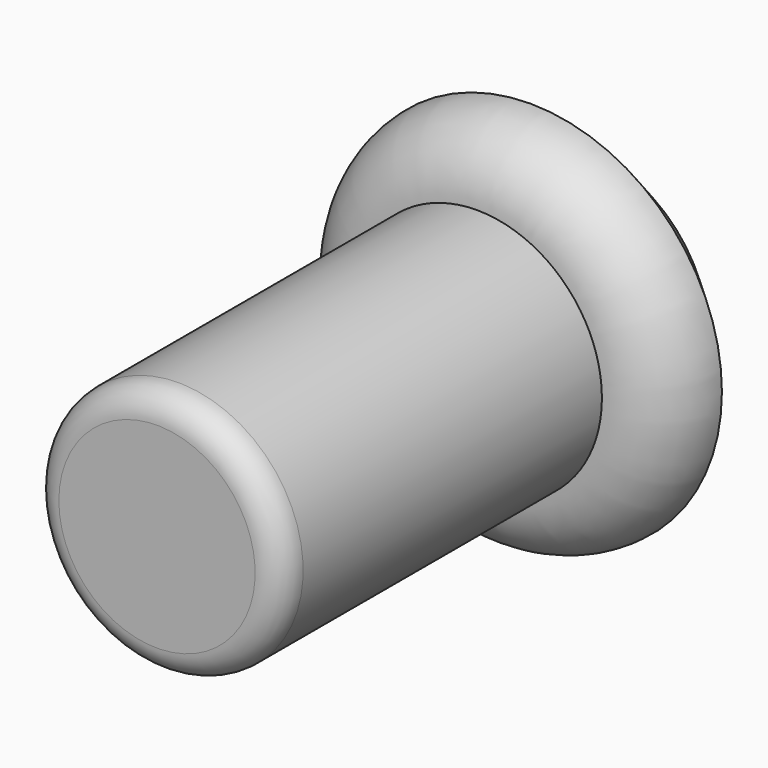
from build123d import *

# Parameters (mm, degrees)
F1_R     = 36.4721508719
F2_DEPTH = 25.399999693
F3_SIZE  = 12.7
F4_R     = 12.69999
F5_R     = 23.7721508719
F6_DEPTH = 101.6
F7_R     = 5.08


# Not quite as in the source:
# - a fillet or chamfer is up to 0.001 mm smaller than in the source, because OpenCascade refuses the exact size


with BuildPart() as f2:
    # F1 (on face) → F2 (new body)
    with BuildSketch(Plane.XZ):
        with Locations((27.7979820967, -14.2051279545)):
            Circle(F1_R)
    extrude(amount=-F2_DEPTH)

    # F3
    f3_edges = [f2.edges().sort_by_distance(p)[0] for p in [
        (-8.674169, 25.4, -14.205128),
    ]]
    chamfer(f3_edges, length=F3_SIZE)

    # F4 (radius 12.7 in the source; OpenCascade refuses exactly that, so slightly less here)
    f4_edges = [f2.edges().sort_by_distance(p)[0] for p in [
        (-8.674169, 0, -14.205128),
    ]]
    fillet(f4_edges, radius=F4_R)

    # F5 (on face) → F6 (join)
    with BuildSketch(Plane(origin=(0, 25.399999693, 0), x_dir=(-1, 0, 0), z_dir=(0, 1, 0))):
        with Locations((-27.7979820967, -14.2051279545)):
            Circle(F5_R)
    extrude(amount=-F6_DEPTH)

    # F7
    f7_edges = [f2.edges().sort_by_distance(p)[0] for p in [
        (51.570133, -76.2, -14.205128),
    ]]
    fillet(f7_edges, radius=F7_R)


solid = f2.part
